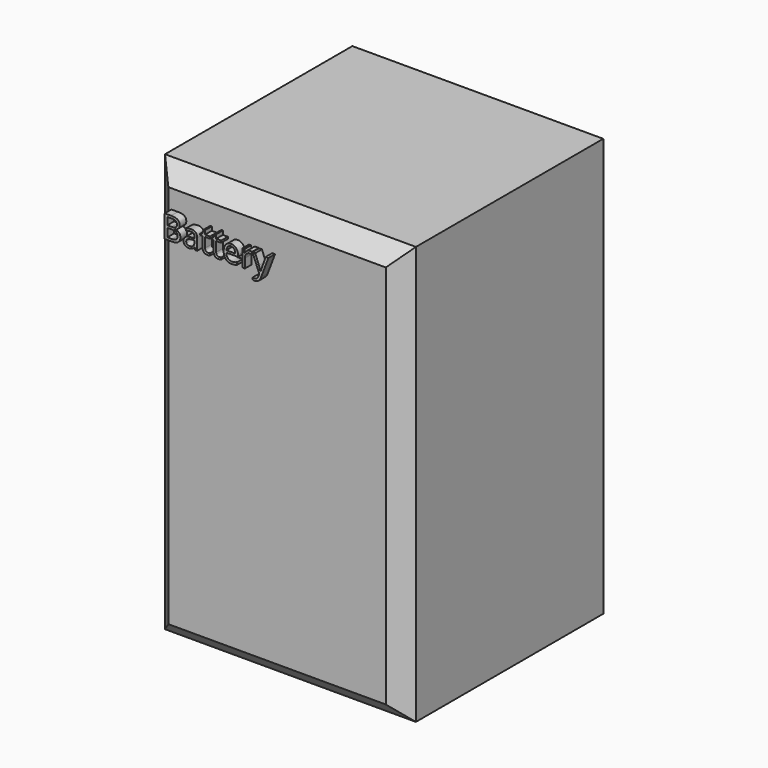
from build123d import *

# Parameters (mm, degrees)
F0_W         = 76.2
F0_H         = 127
F1_DEPTH     = 76.2
F2_SIZE      = 5.08
F3_TEXT_SIZE = 9.5788233161
F4_DEPTH     = 2.54


# Not quite as in the source:
# - Text() gives the source's letters only with a copy of the font that has no kerning and outlines rounded to 1/6400 em; it was checked with that copy


with BuildPart() as f1:
    # F0 (on Front) → F1 (new body)
    with BuildSketch(Plane.XZ):
        Rectangle(F0_W, F0_H)
    extrude(amount=F1_DEPTH)

    # F2
    f2_edges = [f1.edges().sort_by_distance(p)[0] for p in [
        (38.1, -76.2, 0),
        (0, -76.2, 63.5),
        (-38.1, -76.2, 0),
        (0, -76.2, -63.5),
    ]]
    chamfer(f2_edges, length=F2_SIZE)

    # F3 (on face) → F4 (join)
    with BuildSketch(Plane.XZ.offset(76.2)):
        with Locations((-33.02, 45.9103100384)):
            Text('Battery', F3_TEXT_SIZE, font='Open Sans', text_align=(TextAlign.LEFT, TextAlign.BOTTOM))
    extrude(amount=F4_DEPTH)


solid = f1.part
